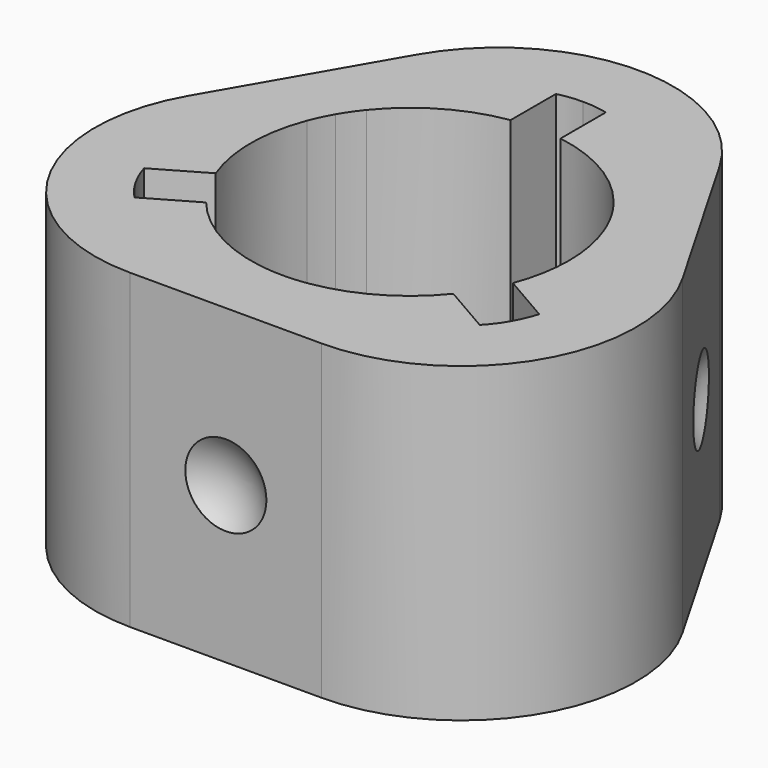
from build123d import *

# Parameters (mm, degrees)
F1_DEPTH        = 25
F2_W            = 2
F2_H            = 1.5
F3_DEPTH        = 16
F6_COPIES_COUNT = 3


# Not quite as in the source:
# - a pattern or mirror of a feature is missing from the dataset's text; its kind, count and spacing are read off the source's solid


with BuildPart() as f1:
    # F0 (on Top) → F1 (new body)
    with BuildSketch(Plane.XY):
        with BuildLine():
            ThreePointArc((7.6794919243, -4), (19.8038475773, 3), (19.8038475773, 17))
            Line((19.8038475773, 17), (12.124355653, 30.3012701892))
            ThreePointArc((12.124355653, 30.3012701892), (0, 37.3012701892), (-12.124355653, 30.3012701892))
            Line((-12.124355653, 30.3012701892), (-19.8038475773, 17))
            ThreePointArc((-19.8038475773, 17), (-19.8038475773, 3), (-7.6794919243, -4))
            Line((-7.6794919243, -4), (0, -4))
            Line((0, -4), (7.6794919243, -4))
        make_face()
        with BuildLine():
            Line((7.6794919243, 0), (0, 0))
            Line((0, 0), (-7.6794919243, 0))
            ThreePointArc((-7.6794919243, 0), (-16.3397459622, 5), (-16.3397459622, 15))
            Line((-16.3397459622, 15), (-8.6602540378, 28.3012701892))
            ThreePointArc((-8.6602540378, 28.3012701892), (0, 33.3012701892), (8.6602540378, 28.3012701892))
            Line((8.6602540378, 28.3012701892), (16.3397459622, 15))
            ThreePointArc((16.3397459622, 15), (16.3397459622, 5), (7.6794919243, 0))
        make_face(mode=Mode.SUBTRACT)
    extrude(amount=F1_DEPTH)

    # F2 (on face) → F3 (join)
    with BuildSketch(Plane.XY.offset(25)):
        Polygon((-11.5, 23.3826859022), (-12.5, 21.6506350946), (-11.2009618943, 20.9006350946), (-10.2009618943, 22.6326859022), align=None)
        Polygon((-11.2009618943, 20.9006350946), (-12.5, 21.6506350946), (-13.5, 19.918584287), (-12.2009618943, 19.168584287), align=None)
        with BuildLine():
            Line((16.3397459622, 5), (15.0407078565, 5.75))
            ThreePointArc((15.0407078565, 5.75), (14.4853104046, 4.9077672075), (13.8340359349, 4.137271282))
            Line((13.8340359349, 4.137271282), (15.1647732985, 3.3689697069))
            ThreePointArc((15.1647732985, 3.3689697069), (15.7933469507, 4.1548860909), (16.3397459622, 5))
        make_face()
        with BuildLine():
            ThreePointArc((15.8340359349, 7.6013728971), (15.4924041247, 6.6521046987), (15.0407078565, 5.75))
            Line((15.0407078565, 5.75), (16.3397459622, 5))
            ThreePointArc((16.3397459622, 5), (16.7984365708, 5.895752379), (17.1647732985, 6.833071322))
            Line((17.1647732985, 6.833071322), (15.8340359349, 7.6013728971))
        make_face()
        Polygon((12.5, 21.6506350946), (11.2009618943, 20.9006350946), (12.2009618943, 19.168584287), (13.5, 19.918584287), align=None)
        Polygon((10.2009618943, 22.6326859022), (11.2009618943, 20.9006350946), (12.5, 21.6506350946), (11.5, 23.3826859022), align=None)
        with BuildLine():
            Line((-15.8340359349, 7.6013728971), (-17.1647732985, 6.833071322))
            ThreePointArc((-17.1647732985, 6.833071322), (-16.7984365708, 5.895752379), (-16.3397459622, 5))
            Line((-16.3397459622, 5), (-15.0407078565, 5.75))
            ThreePointArc((-15.0407078565, 5.75), (-15.4924041247, 6.6521046987), (-15.8340359349, 7.6013728971))
        make_face()
        with BuildLine():
            Line((-15.0407078565, 5.75), (-16.3397459622, 5))
            ThreePointArc((-16.3397459622, 5), (-15.7933469507, 4.1548860909), (-15.1647732985, 3.3689697069))
            Line((-15.1647732985, 3.3689697069), (-13.8340359349, 4.137271282))
            ThreePointArc((-13.8340359349, 4.137271282), (-14.4853104046, 4.9077672075), (-15.0407078565, 5.75))
        make_face()
        with BuildLine():
            Line((-8.6602540378, 28.3012701892), (-11.5, 23.3826859022))
            Line((-11.5, 23.3826859022), (-10.2009618943, 22.6326859022))
            Line((-10.2009618943, 22.6326859022), (-7.3612159322, 27.5512701892))
            ThreePointArc((-7.3612159322, 27.5512701892), (-5.0922327925, 30.1070886696), (-2, 31.5626260102))
            Line((-2, 31.5626260102), (-2, 33.0992291604))
            ThreePointArc((-2, 33.0992291604), (-5.8451139091, 31.4151252157), (-8.6602540378, 28.3012701892))
        make_face()
        with BuildLine():
            Line((-12.2009618943, 19.168584287), (-13.5, 19.918584287))
            Line((-13.5, 19.918584287), (-16.3397459622, 15))
            ThreePointArc((-16.3397459622, 15), (-17.6288534544, 11.0050896201), (-17.1647732985, 6.833071322))
            Line((-17.1647732985, 6.833071322), (-15.8340359349, 7.6013728971))
            ThreePointArc((-15.8340359349, 7.6013728971), (-16.1196200181, 11.0070937201), (-15.0407078565, 14.25))
            Line((-15.0407078565, 14.25), (-12.2009618943, 19.168584287))
        make_face()
        with BuildLine():
            Line((-13.8340359349, 4.137271282), (-15.1647732985, 3.3689697069))
            ThreePointArc((-15.1647732985, 3.3689697069), (-11.7837395453, 0.8810553535), (-7.6794919243, 0))
            Line((-7.6794919243, 0), (-2, 0))
            Line((-2, 0), (-2, 1.5))
            Line((-2, 1.5), (-7.6794919243, 1.5))
            ThreePointArc((-7.6794919243, 1.5), (-11.0273872256, 2.1870877996), (-13.8340359349, 4.137271282))
        make_face()
        with Locations((-1, 0.75)):
            Rectangle(F2_W, F2_H)
        with Locations((1, 0.75)):
            Rectangle(F2_W, F2_H)
        with BuildLine():
            Line((15.1647732985, 3.3689697069), (13.8340359349, 4.137271282))
            ThreePointArc((13.8340359349, 4.137271282), (11.0273872256, 2.1870877996), (7.6794919243, 1.5))
            Line((7.6794919243, 1.5), (2, 1.5))
            Line((2, 1.5), (2, 0))
            Line((2, 0), (7.6794919243, 0))
            ThreePointArc((7.6794919243, 0), (11.7837395453, 0.8810553535), (15.1647732985, 3.3689697069))
        make_face()
        with BuildLine():
            ThreePointArc((15.0407078565, 14.25), (16.1196200181, 11.0070937201), (15.8340359349, 7.6013728971))
            Line((15.8340359349, 7.6013728971), (17.1647732985, 6.833071322))
            ThreePointArc((17.1647732985, 6.833071322), (17.6288534544, 11.0050896201), (16.3397459622, 15))
            Line((16.3397459622, 15), (13.5, 19.918584287))
            Line((13.5, 19.918584287), (12.2009618943, 19.168584287))
            Line((12.2009618943, 19.168584287), (15.0407078565, 14.25))
        make_face()
        with BuildLine():
            ThreePointArc((8.6602540378, 28.3012701892), (5.8451139091, 31.4151252157), (2, 33.0992291604))
            Line((2, 33.0992291604), (2, 31.5626260102))
            ThreePointArc((2, 31.5626260102), (5.0922327925, 30.1070886696), (7.3612159322, 27.5512701892))
            Line((7.3612159322, 27.5512701892), (10.2009618943, 22.6326859022))
            Line((10.2009618943, 22.6326859022), (11.5, 23.3826859022))
            Line((11.5, 23.3826859022), (8.6602540378, 28.3012701892))
        make_face()
        with BuildLine():
            ThreePointArc((2, 33.0992291604), (1.0050896201, 33.2506317193), (0, 33.3012701892))
            Line((0, 33.3012701892), (0, 31.8012701892))
            ThreePointArc((0, 31.8012701892), (1.0070937201, 31.741398283), (2, 31.5626260102))
            Line((2, 31.5626260102), (2, 33.0992291604))
        make_face()
        with BuildLine():
            ThreePointArc((0, 33.3012701892), (-1.0050896201, 33.2506317193), (-2, 33.0992291604))
            Line((-2, 33.0992291604), (-2, 31.5626260102))
            ThreePointArc((-2, 31.5626260102), (-1.0070937201, 31.741398283), (0, 31.8012701892))
            Line((0, 31.8012701892), (0, 33.3012701892))
        make_face()
        with BuildLine():
            Line((-11.9051306732, 18.9977860519), (-12.2009618943, 19.168584287))
            Line((-12.2009618943, 19.168584287), (-15.0407078565, 14.25))
            ThreePointArc((-15.0407078565, 14.25), (-16.1196200181, 11.0070937201), (-15.8340359349, 7.6013728971))
            Line((-15.8340359349, 7.6013728971), (-11.9051306732, 9.8697274076))
            ThreePointArc((-11.9051306732, 9.8697274076), (-12.75, 14.4337567297), (-11.9051306732, 18.9977860519))
        make_face()
        with BuildLine():
            ThreePointArc((-2, 1.8415964703), (-6.375, 3.3919328315), (-9.9051306732, 6.4056257924))
            Line((-9.9051306732, 6.4056257924), (-13.8340359349, 4.137271282))
            ThreePointArc((-13.8340359349, 4.137271282), (-11.0273872256, 2.1870877996), (-7.6794919243, 1.5))
            Line((-7.6794919243, 1.5), (-2, 1.5))
            Line((-2, 1.5), (-2, 1.8415964703))
        make_face()
        with BuildLine():
            Line((13.8340359349, 4.137271282), (9.9051306732, 6.4056257924))
            ThreePointArc((9.9051306732, 6.4056257924), (6.375, 3.3919328315), (2, 1.8415964703))
            Line((2, 1.8415964703), (2, 1.5))
            Line((2, 1.5), (7.6794919243, 1.5))
            ThreePointArc((7.6794919243, 1.5), (11.0273872256, 2.1870877996), (13.8340359349, 4.137271282))
        make_face()
        with BuildLine():
            ThreePointArc((12.75, 14.4337567297), (12.5370035512, 12.1129719577), (11.9051306732, 9.8697274076))
            Line((11.9051306732, 9.8697274076), (15.8340359349, 7.6013728971))
            ThreePointArc((15.8340359349, 7.6013728971), (16.1196200181, 11.0070937201), (15.0407078565, 14.25))
            Line((15.0407078565, 14.25), (12.2009618943, 19.168584287))
            Line((12.2009618943, 19.168584287), (11.9051306732, 18.9977860519))
            ThreePointArc((11.9051306732, 18.9977860519), (12.5370035512, 16.7545415018), (12.75, 14.4337567297))
        make_face()
        with BuildLine():
            ThreePointArc((2, 27.0259169892), (6.375, 25.475580628), (9.9051306732, 22.461887667))
            Line((9.9051306732, 22.461887667), (10.2009618943, 22.6326859022))
            Line((10.2009618943, 22.6326859022), (7.3612159322, 27.5512701892))
            ThreePointArc((7.3612159322, 27.5512701892), (5.0922327925, 30.1070886696), (2, 31.5626260102))
            Line((2, 31.5626260102), (2, 27.0259169892))
        make_face()
        with BuildLine():
            Line((-7.3612159322, 27.5512701892), (-10.2009618943, 22.6326859022))
            Line((-10.2009618943, 22.6326859022), (-9.9051306732, 22.461887667))
            ThreePointArc((-9.9051306732, 22.461887667), (-6.375, 25.475580628), (-2, 27.0259169892))
            Line((-2, 27.0259169892), (-2, 31.5626260102))
            ThreePointArc((-2, 31.5626260102), (-5.0922327925, 30.1070886696), (-7.3612159322, 27.5512701892))
        make_face()
        with BuildLine():
            Line((-10.2009618943, 22.6326859022), (-11.2009618943, 20.9006350946))
            Line((-11.2009618943, 20.9006350946), (-11.0418238983, 20.8087567297))
            ThreePointArc((-11.0418238983, 20.8087567297), (-10.5060428768, 21.6577143065), (-9.9051306732, 22.461887667))
            Line((-9.9051306732, 22.461887667), (-10.2009618943, 22.6326859022))
        make_face()
        with BuildLine():
            Line((-11.0418238983, 20.8087567297), (-11.2009618943, 20.9006350946))
            Line((-11.2009618943, 20.9006350946), (-12.2009618943, 19.168584287))
            Line((-12.2009618943, 19.168584287), (-11.9051306732, 18.9977860519))
            ThreePointArc((-11.9051306732, 18.9977860519), (-11.5091522157, 19.9202779659), (-11.0418238983, 20.8087567297))
        make_face()
        with BuildLine():
            ThreePointArc((9.9051306732, 22.461887667), (10.5060428768, 21.6577143065), (11.0418238983, 20.8087567297))
            Line((11.0418238983, 20.8087567297), (11.2009618943, 20.9006350946))
            Line((11.2009618943, 20.9006350946), (10.2009618943, 22.6326859022))
            Line((10.2009618943, 22.6326859022), (9.9051306732, 22.461887667))
        make_face()
        with BuildLine():
            Line((11.2009618943, 20.9006350946), (11.0418238983, 20.8087567297))
            ThreePointArc((11.0418238983, 20.8087567297), (11.5091522157, 19.9202779659), (11.9051306732, 18.9977860519))
            Line((11.9051306732, 18.9977860519), (12.2009618943, 19.168584287))
            Line((12.2009618943, 19.168584287), (11.2009618943, 20.9006350946))
        make_face()
        with BuildLine():
            ThreePointArc((2, 1.8415964703), (1.003109339, 1.7232779168), (0, 1.6837567297))
            Line((0, 1.6837567297), (0, 1.5))
            Line((0, 1.5), (2, 1.5))
            Line((2, 1.5), (2, 1.8415964703))
        make_face()
        with BuildLine():
            Line((0, 1.5), (0, 1.6837567297))
            ThreePointArc((0, 1.6837567297), (-1.003109339, 1.7232779168), (-2, 1.8415964703))
            Line((-2, 1.8415964703), (-2, 1.5))
            Line((-2, 1.5), (0, 1.5))
        make_face()
    extrude(amount=-F3_DEPTH)

    # F5 (on offset) → F6 (revolve, cut)
    with BuildSketch(Plane.XY.offset(12.5)):
        with BuildLine():
            ThreePointArc((0, -12.8), (3.5355339059, -11.3355339059), (5, -7.8))
            ThreePointArc((5, -7.8), (3.5355339059, -4.2644660941), (0, -2.8))
            Line((0, -2.8), (0, -12.8))
        make_face()
    f6 = revolve(axis=Axis((0, -7.8, 12.5), (0, 1, 0)), mode=Mode.SUBTRACT)

    # F6_copies: F6 ×3 about axis
    f6_copies_axis = Axis((0, 14.433757, 0), (0, 0, 1))
    for i in range(1, F6_COPIES_COUNT):
        add(f6.rotate(f6_copies_axis, i * 360 / F6_COPIES_COUNT), mode=Mode.SUBTRACT)


solid = f1.part
